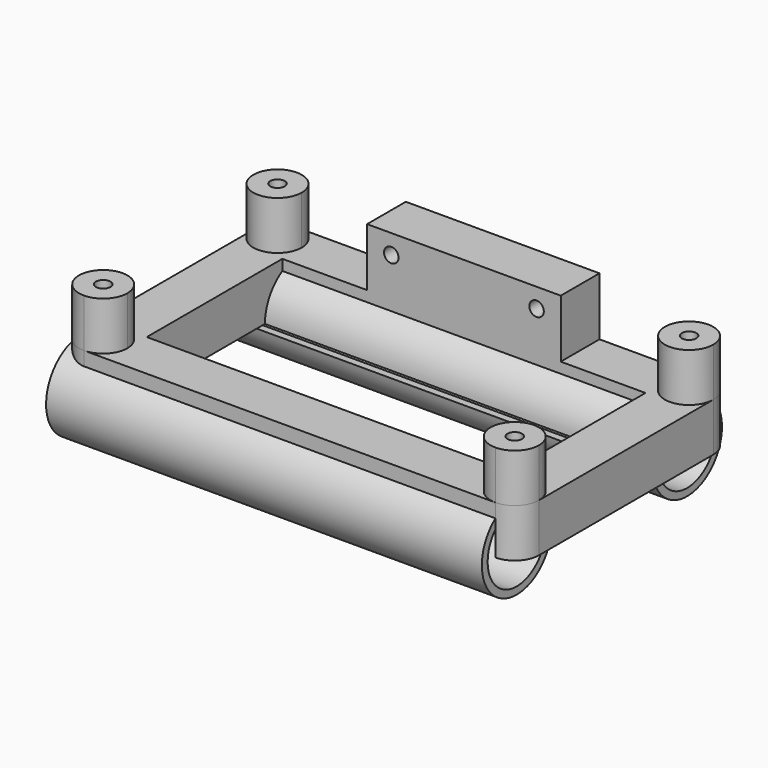
from build123d import *
from build123d import SkipClean  # not in build123d's __all__

# Parameters (mm, degrees)
F0_W      = 95
F0_H      = 55
F0_W_2    = 75
F0_H_2    = 35
F1_DEPTH  = 10
F2_R      = 5
F3_W      = 40
F3_H      = 10
F4_DEPTH  = 12
F5_R      = 1.5
F6_DEPTH  = 25
F7_W      = 6
F7_H      = 5
F7_R      = 1.5
F8_DEPTH  = 5
F9_R      = 1
F10_R     = 9
F10_R_2   = 7.5
F11_DEPTH = 90
F13_DEPTH = 90
F14_R     = 1.5
F15_DEPTH = 10


with BuildPart() as f1:
    # F0 (on Top) → F1 (new body)
    with BuildSketch(Plane.XY):
        Rectangle(F0_W, F0_H)
        Rectangle(F0_W_2, F0_H_2, mode=Mode.SUBTRACT)
    extrude(amount=F1_DEPTH)

    # F2
    f2_edges = [f1.edges().sort_by_distance(p)[0] for p in [
        (-47.5, -27.5, 5),
        (47.5, -27.5, 5),
        (47.5, 27.5, 5),
        (-47.5, 27.5, 5),
    ]]
    fillet(f2_edges, radius=F2_R)

    # F3 (on face) → F4 (join)
    with BuildSketch(Plane.XY.offset(10)):
        with Locations((0, 22.5)):
            Rectangle(F3_W, F3_H)
    extrude(amount=F4_DEPTH)

    # F5 (on face) → F6 (cut)
    with BuildSketch(Plane.XZ.offset(-17.5)):
        with Locations((-15, 18)):
            Circle(F5_R)
        with Locations((15, 18)):
            Circle(F5_R)
    extrude(amount=-F6_DEPTH, mode=Mode.SUBTRACT)

    # F7 (on face) → F8 (cut)
    with BuildSketch(Plane(origin=(0, 27.5, 0), x_dir=(-1, 0, 0), z_dir=(0, 1, 0))):
        with Locations((15, 18)):
            Rectangle(F7_W, F7_H)
        with Locations((15, 18)):
            Circle(F7_R, mode=Mode.SUBTRACT)
        with Locations((-15, 18)):
            Rectangle(F7_W, F7_H)
        with Locations((-15, 18)):
            Circle(F7_R, mode=Mode.SUBTRACT)
    extrude(amount=-F8_DEPTH, mode=Mode.SUBTRACT)

    # F9
    f9_edges = [f1.edges().sort_by_distance(p)[0] for p in [
        (18, 25, 20.5),
        (12, 25, 20.5),
        (18, 25, 15.5),
        (12, 25, 15.5),
        (-18, 25, 20.5),
        (-12, 25, 20.5),
        (-12, 25, 15.5),
        (-18, 25, 15.5),
    ]]
    fillet(f9_edges, radius=F9_R)

    # F10 (on face) → F11 (join)
    with BuildSketch(Plane(origin=(-47.5, 0, 0), x_dir=(0, -1, 0), z_dir=(-1, 0, 0))):
        with BuildLine():
            ThreePointArc((31, 0), (22, 9), (13, 0))
            ThreePointArc((13, 0), (22, -9), (31, 0))
        make_face()
        with BuildLine():
            ThreePointArc((29.5, 0), (22, -7.5), (14.5, 0))
            ThreePointArc((14.5, 0), (22, 7.5), (29.5, 0))
        make_face(mode=Mode.SUBTRACT)
        with Locations((-22, 0)):
            Circle(F10_R)
        with Locations((-22, 0)):
            Circle(F10_R_2, mode=Mode.SUBTRACT)
    extrude(amount=-F11_DEPTH)

    # F12 (on face) → F13 (cut)
    with BuildSketch(Plane(origin=(-47.5, 0, 0), x_dir=(0, -1, 0), z_dir=(-1, 0, 0))):
        with BuildLine():
            Line((-15.325489454, 0), (-14.5, 0))
            ThreePointArc((-14.5, 0), (-16.876524617, 5.4772255751), (-22.5, 7.4833147735))
            Line((-22.5, 7.4833147735), (-22.5, 0))
            Line((-22.5, 0), (-15.325489454, 0))
        make_face()
        with BuildLine():
            Line((-14.5, -1.5), (-14.5, 0))
            ThreePointArc((-14.5, 0), (-14.5379788525, -0.753817215), (-14.6515307717, -1.5))
            Line((-14.6515307717, -1.5), (-14.5, -1.5))
        make_face()
        with BuildLine():
            ThreePointArc((22.5, 7.4833147735), (16.876524617, 5.4772255751), (14.5, 0))
            Line((14.5, 0), (15.7362241298, 0))
            Line((15.7362241298, 0), (22.5, 0))
            Line((22.5, 0), (22.5, 7.4833147735))
        make_face()
        with BuildLine():
            ThreePointArc((14.6515307717, -1.5), (14.5379788525, -0.753817215), (14.5, 0))
            Line((14.5, 0), (14.5, -1.5))
            Line((14.5, -1.5), (14.6515307717, -1.5))
        make_face()
        with BuildLine():
            Line((15.7362241298, 0), (14.5, 0))
            ThreePointArc((14.5, 0), (14.5379788525, -0.753817215), (14.6515307717, -1.5))
            Line((14.6515307717, -1.5), (15.7362241298, -1.5))
            Line((15.7362241298, -1.5), (15.7362241298, 0))
        make_face()
        with BuildLine():
            Line((14.5, 0), (13, 0))
            ThreePointArc((13, 0), (13.0315252949, -0.7526363425), (13.1258803254, -1.5))
            Line((13.1258803254, -1.5), (14.5, -1.5))
            Line((14.5, -1.5), (14.5, 0))
        make_face()
        with BuildLine():
            Line((-13, 0), (-14.5, 0))
            Line((-14.5, 0), (-14.5, -1.5))
            Line((-14.5, -1.5), (-13.1258803254, -1.5))
            ThreePointArc((-13.1258803254, -1.5), (-13.0315252949, -0.7526363425), (-13, 0))
        make_face()
        with BuildLine():
            Line((-22.5, 0), (-22.5, 7.4833147735))
            ThreePointArc((-22.5, 7.4833147735), (-27.6480411448, -4.9345345502), (-14.6515307717, -1.5))
            Line((-14.6515307717, -1.5), (-15.325489454, -1.5))
            Line((-15.325489454, -1.5), (-15.325489454, 0))
            Line((-15.325489454, 0), (-22.5, 0))
        make_face()
        with BuildLine():
            ThreePointArc((29.5, 0), (27.4772255751, 5.123475383), (22.5, 7.4833147735))
            Line((22.5, 7.4833147735), (22.5, 0))
            Line((22.5, 0), (15.7362241298, 0))
            Line((15.7362241298, 0), (15.7362241298, -1.5))
            Line((15.7362241298, -1.5), (14.6515307717, -1.5))
            ThreePointArc((14.6515307717, -1.5), (22.753817215, -7.4620211475), (29.5, 0))
        make_face()
    extrude(amount=-F13_DEPTH, mode=Mode.SUBTRACT)

    # F14 (on face) → F15 (join)
    with BuildSketch(Plane.XY.offset(10)):
        with BuildLine():
            ThreePointArc((-42.5, 27.5), (-46.0355339059, 26.0355339059), (-47.5, 22.5))
            ThreePointArc((-47.5, 22.5), (-42.5, 17.5), (-37.5, 22.5))
            ThreePointArc((-37.5, 22.5), (-38.9644660941, 26.0355339059), (-42.5, 27.5))
        make_face()
        with Locations((-42.5, 22.5)):
            Circle(F14_R, mode=Mode.SUBTRACT)
        with BuildLine():
            ThreePointArc((-42.5, -27.5), (-38.9644660941, -26.0355339059), (-37.5, -22.5))
            ThreePointArc((-37.5, -22.5), (-42.5, -17.5), (-47.5, -22.5))
            ThreePointArc((-47.5, -22.5), (-46.0355339059, -26.0355339059), (-42.5, -27.5))
        make_face()
        with Locations((-42.5, -22.5)):
            Circle(F14_R, mode=Mode.SUBTRACT)
        with BuildLine():
            ThreePointArc((47.5, -22.5), (38.9644660941, -18.9644660941), (42.5, -27.5))
            ThreePointArc((42.5, -27.5), (46.0355339059, -26.0355339059), (47.5, -22.5))
        make_face()
        with Locations((42.5, -22.5)):
            Circle(F14_R, mode=Mode.SUBTRACT)
        with BuildLine():
            ThreePointArc((42.5, 27.5), (38.9644660941, 18.9644660941), (47.5, 22.5))
            ThreePointArc((47.5, 22.5), (46.0355339059, 26.0355339059), (42.5, 27.5))
        make_face()
        with Locations((42.5, 22.5)):
            Circle(F14_R, mode=Mode.SUBTRACT)
    with SkipClean():  # cleaning this boolean's faces spoils the solid; the shape is the same uncleaned
        extrude(amount=F15_DEPTH)


solid = f1.part
